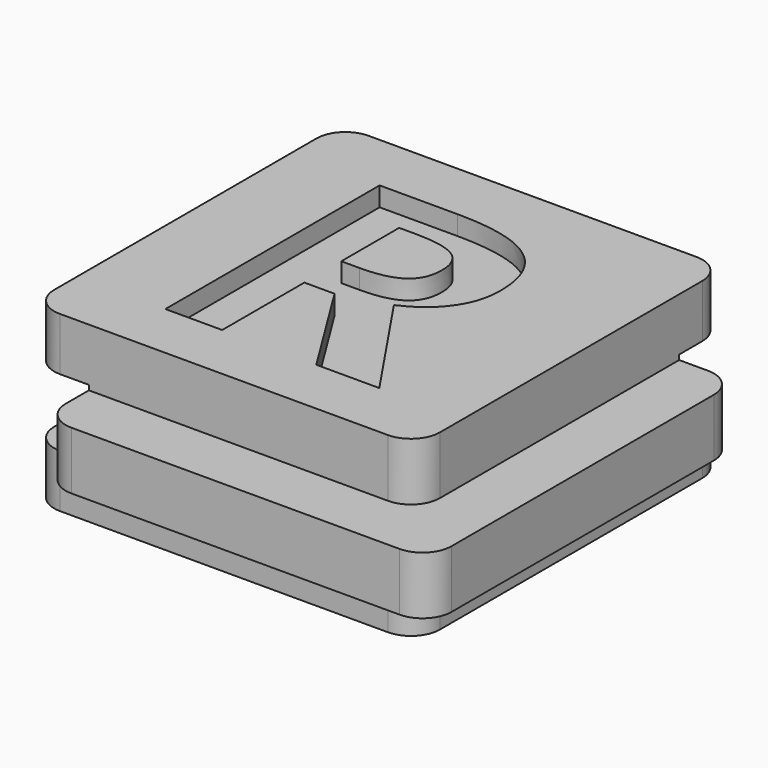
from build123d import *

# Parameters (mm, degrees)
F0_W         = 14
F0_H         = 3
F0_W_2       = 3
F1_DEPTH     = 20
F2_DEPTH     = 3
F3_W         = 3
F3_H         = 3
F4_DEPTH     = 100
F5_W         = 3
F5_H         = 3.5
F6_DEPTH     = 100
F7_R         = 1.5
F8_TEXT_SIZE = 19.4444444444
F9_DEPTH     = 1


# Not quite as in the source:
# - Text() gives the source's letters only with a copy of the font that has no kerning and outlines rounded to 1/6400 em; it was checked with that copy


with BuildPart() as f1:
    # F0 (on Front) → F1 (new body)
    with BuildSketch(Plane.XZ):
        Polygon((10, 1.5), (10, 4.5), (-10, 4.5), (-10, 1.5), (-7, 1.5), (7, 1.5), align=None)
        Rectangle(F0_W, F0_H)
        with Locations((11.5, 0)):
            Rectangle(F0_W_2, F0_H)
        with Locations((8.5, 0)):
            Rectangle(F0_W_2, F0_H)
        with Locations((-8.5, 0)):
            Rectangle(F0_W_2, F0_H)
        Polygon((10, -4.5), (10, -1.5), (7, -1.5), (-7, -1.5), (-10, -1.5), (-10, -4.5), align=None)
    extrude(amount=-F1_DEPTH)

    # F0 (on Front) → F2 (join)
    with BuildSketch(Plane.XZ):
        with Locations((-8.5, 0)):
            Rectangle(F0_W_2, F0_H)
        Rectangle(F0_W, F0_H)
        with Locations((8.5, 0)):
            Rectangle(F0_W_2, F0_H)
        with Locations((11.5, 0)):
            Rectangle(F0_W_2, F0_H)
    extrude(amount=F2_DEPTH)

    # F3 (on face) → F4 (cut)
    with BuildSketch(Plane.YZ.offset(13)):
        Polygon((23, -1.75), (23, 1.75), (17, 1.75), (17, 1.5), (20, 1.5), (20, -1.5), (17, -1.5), (17, -1.75), align=None)
        with Locations((18.5, 0)):
            Rectangle(F3_W, F3_H)
    extrude(amount=-F4_DEPTH, mode=Mode.SUBTRACT)

    # F5 (on face) → F6 (cut)
    with BuildSketch(Plane(origin=(0, 17, 0), x_dir=(-1, 0, 0), z_dir=(0, 1, 0))):
        with Locations((11.5, 0)):
            Rectangle(F5_W, F5_H)
        with Locations((8.5, 0)):
            Rectangle(F5_W, F5_H)
    extrude(amount=-F6_DEPTH, mode=Mode.SUBTRACT)

    # F7
    f7_edges = [f1.edges().sort_by_distance(p)[0] for p in [
        (-7, -3, 0),
        (13, -3, 0),
        (10, 0, 3),
        (10, 0, -3),
        (-10, 0, -3.125),
        (-10, 0, 3.125),
        (-7, 17, 0),
        (-10, 20, 3.125),
        (-10, 20, -3.125),
        (13, 17, 0),
        (10, 20, 3.125),
        (10, 20, -3.125),
    ]]
    fillet(f7_edges, radius=F7_R)

    # F8 (on face) → F9 (cut)
    with BuildSketch(Plane.XY.offset(4.5)):
        with Locations((-7.1801951318, 3)):
            Text('R', F8_TEXT_SIZE, font='Open Sans', font_style=FontStyle.BOLD, text_align=(TextAlign.LEFT, TextAlign.BOTTOM))
    extrude(amount=-F9_DEPTH, mode=Mode.SUBTRACT)


solid = f1.part
